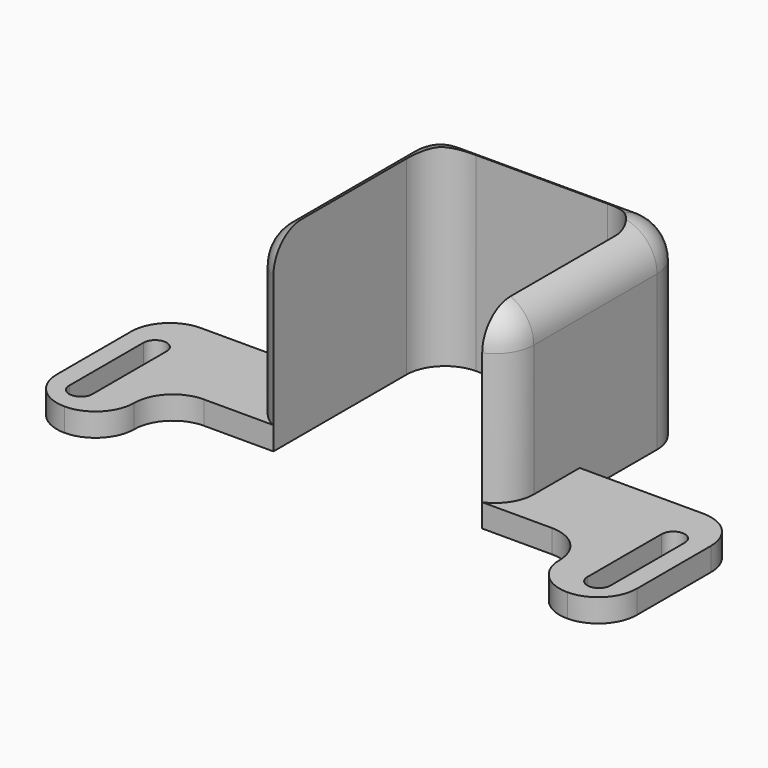
from build123d import *

# Parameters (mm, degrees)
F2_DEPTH     = 25
F3_DEPTH     = 3
F4_DEPTH     = 25
F5_R         = 4.99999
F6_T1_DEPTH  = 25
F6_T3_DEPTH  = 25
F6_T5_DEPTH  = 50
F6_T7_DEPTH  = 33.4564392374
F6_T9_DEPTH  = 50
F6_T11_DEPTH = 33.4564392374
F7_T1_DEPTH  = 19.917424305
F7_T3_DEPTH  = 23
F7_T6_ANGLE  = 89.9999999974
F7_T8_ANGLE  = 89.9999999974
F7_T10_ANGLE = 209.6926070845
F7_T12_ANGLE = 209.6926070845


# Not quite as in the source:
# - a fillet or chamfer that OpenCascade refuses, or shapes differently, is made with other operations: its cross-section is extruded or revolved along the edge and cut away or added
# - a fillet or chamfer is up to 0.001 mm smaller than in the source, because OpenCascade refuses the exact size


with BuildPart() as f2:
    # F0 (on Top) → F2 (new body)
    with BuildSketch(Plane.XY):
        Polygon((16.5, 39.5), (0, 39.5), (-16.5, 39.5), (-16.5, 22), (-16.5, 10), (-13.5, 10), (-13.5, 36.5), (0, 36.5), (13.5, 36.5), (13.5, 10), (16.5, 10), (16.5, 22), align=None)
    extrude(amount=F2_DEPTH)

    # F0 (on Top) → F3 (join)
    with BuildSketch(Plane.XY):
        Polygon((-16.5, 10), (-16.5, 22), (-37.5, 22), (-37.5, 0), (-27.5, 0), (-27.5, 10), align=None)
        Polygon((37.5, 22), (16.5, 22), (16.5, 10), (27.5, 10), (27.5, 0), (37.5, 0), align=None)
    extrude(amount=F3_DEPTH)

    # F1 (on Top) → F4 (cut)
    with BuildSketch(Plane.XY):
        with BuildLine():
            Line((35, 3.8767794613), (35, 15.8767794613))
            ThreePointArc((35, 15.8767794613), (33.5, 17.3767794613), (32, 15.8767794613))
            Line((32, 15.8767794613), (32, 3.8767794613))
            ThreePointArc((32, 3.8767794613), (33.5, 2.3767794613), (35, 3.8767794613))
        make_face()
        with BuildLine():
            ThreePointArc((-32, 15.8767794613), (-33.5, 17.3767794613), (-35, 15.8767794613))
            Line((-35, 15.8767794613), (-35, 3.8767794613))
            ThreePointArc((-35, 3.8767794613), (-33.5, 2.3767794613), (-32, 3.8767794613))
            Line((-32, 3.8767794613), (-32, 15.8767794613))
        make_face()
    extrude(amount=F4_DEPTH, mode=Mode.SUBTRACT)

    # F5 (radius 5 in the source; OpenCascade refuses exactly that, so slightly less here)
    f5_edges = [f2.edges().sort_by_distance(p)[0] for p in [
        (-37.5, 0, 1.5),
        (-27.5, 0, 1.5),
        (-37.5, 22, 1.5),
        (37.5, 22, 1.5),
        (37.5, 0, 1.5),
        (27.5, 0, 1.5),
        (27.5, 10, 1.5),
        (-27.5, 10, 1.5),
    ]]
    fillet(f5_edges, radius=F5_R)

    # F6: fillet of radius 5 on 6 edges, made by hand

    # F6_s2 → F6_t1 (join)
    with BuildSketch(Plane.XY):
        with BuildLine():
            ThreePointArc((13.5, 31.5), (12.0355339059, 35.0355339059), (8.5, 36.5))
            Line((8.5, 36.5), (13.5, 36.5))
            Line((13.5, 36.5), (13.5, 31.5))
        make_face()
    extrude(amount=F6_T1_DEPTH)

    # F6_s4 → F6_t3 (join)
    with BuildSketch(Plane.XY):
        with BuildLine():
            ThreePointArc((-8.5, 36.5), (-12.0355339059, 35.0355339059), (-13.5, 31.5))
            Line((-13.5, 31.5), (-13.5, 36.5))
            Line((-13.5, 36.5), (-8.5, 36.5))
        make_face()
    extrude(amount=F6_T3_DEPTH)

    # F6_s6 → F6_t5 (cut)
    with BuildSketch(Plane.XY.offset(-12.5)):
        with BuildLine():
            ThreePointArc((16.5, 34.5), (15.0355339059, 38.0355339059), (11.5, 39.5))
            Line((11.5, 39.5), (16.5, 39.5))
            Line((16.5, 39.5), (16.5, 34.5))
        make_face()
    extrude(amount=F6_T5_DEPTH, mode=Mode.SUBTRACT)

    # F6_s8 → F6_t7 (cut)
    with BuildSketch(Plane.XY.offset(3)):
        with BuildLine():
            ThreePointArc((13.5, 10), (15.6833001327, 11.8439629074), (16.5, 14.582575695))
            Line((16.5, 14.582575695), (16.5, 10))
            Line((16.5, 10), (13.5, 10))
        make_face()
    extrude(amount=F6_T7_DEPTH, mode=Mode.SUBTRACT)

    # F6_s10 → F6_t9 (cut)
    with BuildSketch(Plane.XY.offset(-12.5)):
        with BuildLine():
            ThreePointArc((-11.5, 39.5), (-15.0355339059, 38.0355339059), (-16.5, 34.5))
            Line((-16.5, 34.5), (-16.5, 39.5))
            Line((-16.5, 39.5), (-11.5, 39.5))
        make_face()
    extrude(amount=F6_T9_DEPTH, mode=Mode.SUBTRACT)

    # F6_s12 → F6_t11 (cut)
    with BuildSketch(Plane.XY.offset(3)):
        with BuildLine():
            ThreePointArc((-13.5, 10), (-15.6833001327, 11.8439629074), (-16.5, 14.582575695))
            Line((-16.5, 14.582575695), (-16.5, 10))
            Line((-16.5, 10), (-13.5, 10))
        make_face()
    extrude(amount=F6_T11_DEPTH, mode=Mode.SUBTRACT)

    # F7: fillet of radius 5 on 3 edges, made by hand

    # F7_s2 → F7_t1 (cut)
    with BuildSketch(Plane.XZ.offset(-34.5)):
        with BuildLine():
            ThreePointArc((-11.5, 25), (-15.0355339059, 23.5355339059), (-16.5, 20))
            Line((-16.5, 20), (-16.5, 25))
            Line((-16.5, 25), (-11.5, 25))
        make_face()
        with BuildLine():
            ThreePointArc((11.5, 25), (15.0355339059, 23.5355339059), (16.5, 20))
            Line((16.5, 20), (16.5, 25))
            Line((16.5, 25), (11.5, 25))
        make_face()
    extrude(amount=F7_T1_DEPTH, mode=Mode.SUBTRACT)

    # F7_s4 → F7_t3 (cut)
    with BuildSketch(Plane.YZ.offset(-11.5)):
        with BuildLine():
            ThreePointArc((34.5, 25), (38.0355339059, 23.5355339059), (39.5, 20))
            Line((39.5, 20), (39.5, 25))
            Line((39.5, 25), (34.5, 25))
        make_face()
    extrude(amount=F7_T3_DEPTH, mode=Mode.SUBTRACT)

    # F7_s5 → F7_t6 (revolve, cut)
    with BuildSketch(Plane.YZ.offset(11.4999999999)):
        with BuildLine():
            ThreePointArc((34.5, 25), (38.0355339059, 23.5355339059), (39.5, 20))
            Line((39.5, 20), (39.5, 25))
            Line((39.5, 25), (34.5, 25))
        make_face()
    revolve(axis=Axis((11.4999999999, 34.4999999999, 25), (0, 0, -1)), revolution_arc=F7_T6_ANGLE, mode=Mode.SUBTRACT)

    # F7_s7 → F7_t8 (revolve, cut)
    with BuildSketch(Plane.XZ.offset(-34.4999999999)):
        with BuildLine():
            ThreePointArc((-11.5, 25), (-15.0355339059, 23.5355339059), (-16.5, 20))
            Line((-16.5, 20), (-16.5, 25))
            Line((-16.5, 25), (-11.5, 25))
        make_face()
    revolve(axis=Axis((-11.4999999999, 34.4999999999, 25), (0, 0, -1)), revolution_arc=F7_T8_ANGLE, mode=Mode.SUBTRACT)

    # F7_s9 → F7_t10 (revolve, cut)
    with BuildSketch(Plane.XZ.offset(-14.5825756948)):
        with BuildLine():
            ThreePointArc((16.5, 20), (15.0355339059, 23.5355339059), (11.5, 25))
            Line((11.5, 25), (16.5, 25))
            Line((16.5, 25), (16.5, 20))
        make_face()
    revolve(axis=Axis((11.5000000002, 14.5825756948, 25), (0, 0, -1)), revolution_arc=F7_T10_ANGLE, mode=Mode.SUBTRACT)

    # F7_s11 → F7_t12 (revolve, cut)
    with BuildSketch(Plane(origin=(-9.0966946013, 15.9529859327, 0), x_dir=(0, 0, 1), z_dir=(-0.4953465841, 0.8686954366, 0))):
        with BuildLine():
            ThreePointArc((25, -2.7665684632), (23.5355339059, 0.7689654427), (20, 2.2334315368))
            Line((20, 2.2334315368), (25, 2.2334315368))
            Line((25, 2.2334315368), (25, -2.7665684632))
        make_face()
    revolve(axis=Axis((-11.5000000002, 14.5825756948, 25), (0, 0, -1)), revolution_arc=F7_T12_ANGLE, mode=Mode.SUBTRACT)


solid = f2.part
